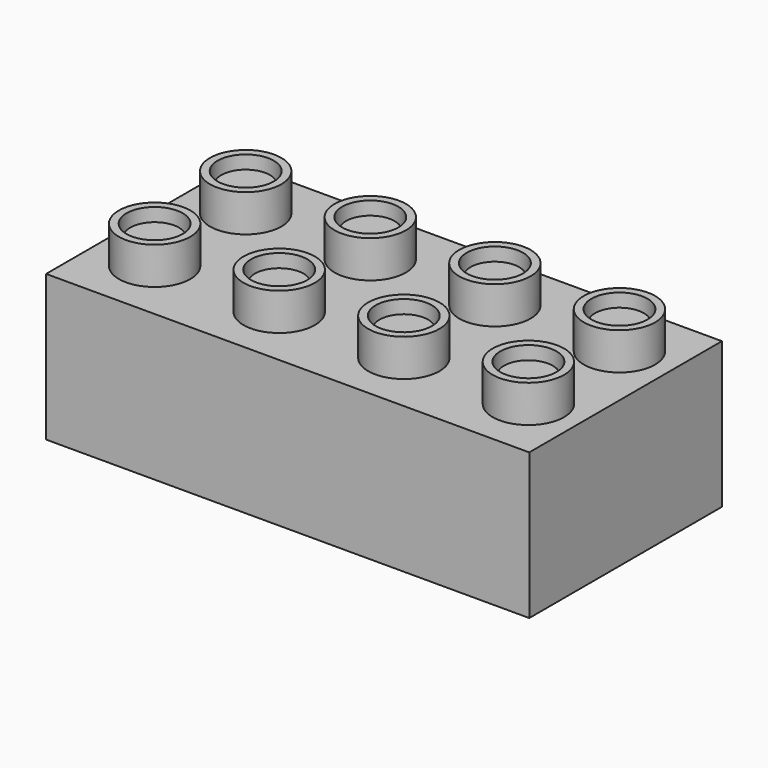
from build123d import *

# Parameters (mm, degrees)
F0_W     = 63.6
F0_H     = 19.2
F1_DEPTH = 15.85
F2_R     = 4.7
F3_DEPTH = 4.9
F4_T     = -2.5
F5_R     = 6.8
F6_DEPTH = 16.5
F7_T     = -1


with BuildPart() as f1:
    # F0 (on Front) → F1 (new body, symmetric)
    with BuildSketch(Plane.XZ):
        with Locations((0, -9.6)):
            Rectangle(F0_W, F0_H)
    extrude(amount=F1_DEPTH, both=True)

    # F2 (on Top) → F3 (join)
    with BuildSketch(Plane.XY):
        with Locations((-24.2, 7.491081953)):
            Circle(F2_R)
        with Locations((-7.8, 7.491081953)):
            Circle(F2_R)
        with Locations((8.6, 7.491081953)):
            Circle(F2_R)
        with Locations((25, 7.491081953)):
            Circle(F2_R)
        with Locations((25, -7.491081953)):
            Circle(F2_R)
        with Locations((8.6, -7.491081953)):
            Circle(F2_R)
        with Locations((-7.8, -7.491081953)):
            Circle(F2_R)
        with Locations((-24.2, -7.491081953)):
            Circle(F2_R)
    extrude(amount=F3_DEPTH)

    # F4
    f4_openings = [f1.faces().sort_by_distance(p)[0] for p in [
        (0, 0, -19.2),
    ]]
    offset(amount=F4_T, openings=f4_openings, kind=Kind.INTERSECTION)

    # F5 (on Top) → F6 (join)
    with BuildSketch(Plane.XY):
        with BuildLine():
            ThreePointArc((9.7, 0), (16.5, -6.8), (23.3, 0))
            ThreePointArc((23.3, 0), (16.5, 6.8), (9.7, 0))
        make_face()
        with Locations((-16.3, 0)):
            Circle(F5_R)
        with BuildLine():
            ThreePointArc((0, -6.7992646661), (4.8728398255, -4.8435524153), (6.9, 0))
            ThreePointArc((6.9, 0), (4.9083261121, 4.8083261121), (0.1, 6.8))
            ThreePointArc((0.1, 6.8), (-4.7083261121, 4.8083261121), (-6.7, 0))
            ThreePointArc((-6.7, 0), (-4.7435524153, -4.7728398255), (0, -6.7992646661))
        make_face()
    extrude(amount=-F6_DEPTH)

    # F7
    f7_openings = [f1.faces().sort_by_distance(p)[0] for p in [
        (16.5, 0, -16.5),
        (0.1, 0, -16.5),
        (-16.3, 0, -16.5),
        (-24.2, -7.491082, 4.9),
        (-24.2, 7.491082, 4.9),
        (-7.8, 7.491082, 4.9),
        (-7.8, -7.491082, 4.9),
        (8.6, -7.491082, 4.9),
        (8.6, 7.491082, 4.9),
        (25, 7.491082, 4.9),
        (25, -7.491082, 4.9),
    ]]
    offset(amount=F7_T, openings=f7_openings, kind=Kind.INTERSECTION)


solid = f1.part
